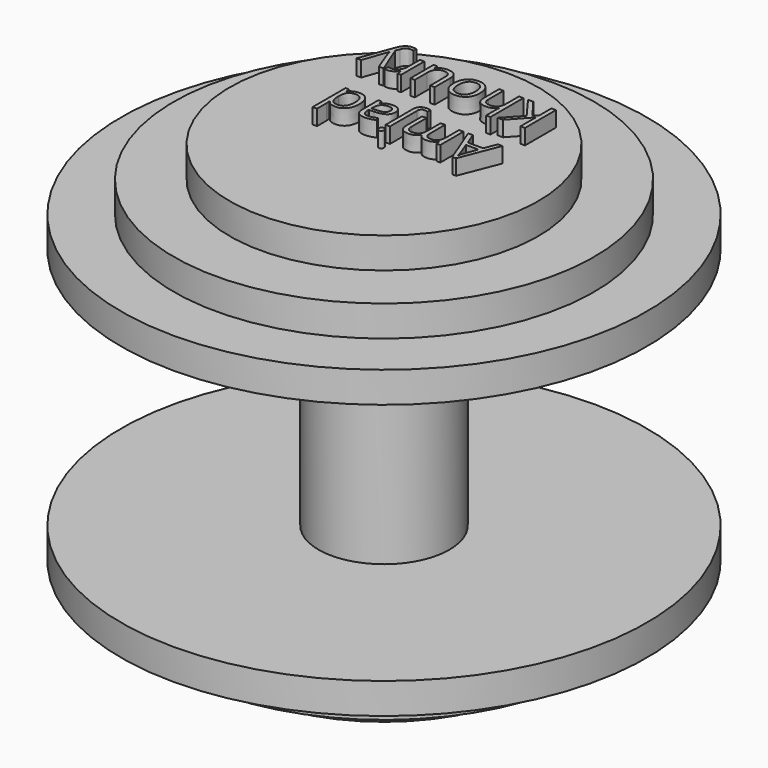
from build123d import *

# Parameters (mm, degrees)
F2_TEXT_SIZE = 5.9242802925
F3_DEPTH     = 2.5
F5_TEXT_SIZE = 8.768324428
F6_DEPTH     = 2.5


# Not quite as in the source:
# - Text() gives the source's letters only with a copy of the font that has no kerning and outlines rounded to 1/6400 em; it was checked with that copy


with BuildPart() as f1:
    # F0 (on Right) → F1 (revolve)
    with BuildSketch(Plane.YZ):
        Polygon((17.606751749, 45.8921257284), (0, 45.8921257284), (0, -23.5071625375), (25, -23.5071625375), (25, -18.5071625375), (34.0583565398, -18.5071625375), (34.0583565398, -13.5071625375), (42.6067408148, -13.5071625375), (42.6067408148, -8.5071625375), (10.6067408148, -8.5071625375), (10.6067408148, 30.8921257284), (42.6067408148, 30.8921257284), (42.6067408148, 35.8921257284), (34.0583565398, 35.8921257284), (34.0583565398, 40.8921257284), (25, 40.8921257284), (25, 45.8921257284), align=None)
    revolve(axis=Axis((0, 0, 11.1924815955), (0, 0, -1)))

    # F2 (on face) → F3 (join)
    with BuildSketch(Plane(origin=(0, 0, -23.5071625375), x_dir=(1, 0, 0), z_dir=(0, 0, -1))):
        with Locations((-14.1933242372, -1.197902179)):
            Text('Much Love', F2_TEXT_SIZE, font='Open Sans', text_align=(TextAlign.LEFT, TextAlign.BOTTOM))
        with Locations((-11.1145498227, -9.2549233768)):
            Text('Reham', F2_TEXT_SIZE, font='Open Sans', text_align=(TextAlign.LEFT, TextAlign.BOTTOM))
    extrude(amount=F3_DEPTH)

    # F5 (on face) → F6 (join)
    with BuildSketch(Plane.XY.offset(45.8921257284)):
        with Locations(Location((15, 5.2238130011), (0, 0, 180))):
            Text('Amjad', F5_TEXT_SIZE, font='Open Sans', text_align=(TextAlign.LEFT, TextAlign.BOTTOM))
        with Locations(Location((15, 17.1487342232), (0, 0, 180))):
            Text('Khoury', F5_TEXT_SIZE, font='Open Sans', text_align=(TextAlign.LEFT, TextAlign.BOTTOM))
    extrude(amount=F6_DEPTH)


solid = f1.part
